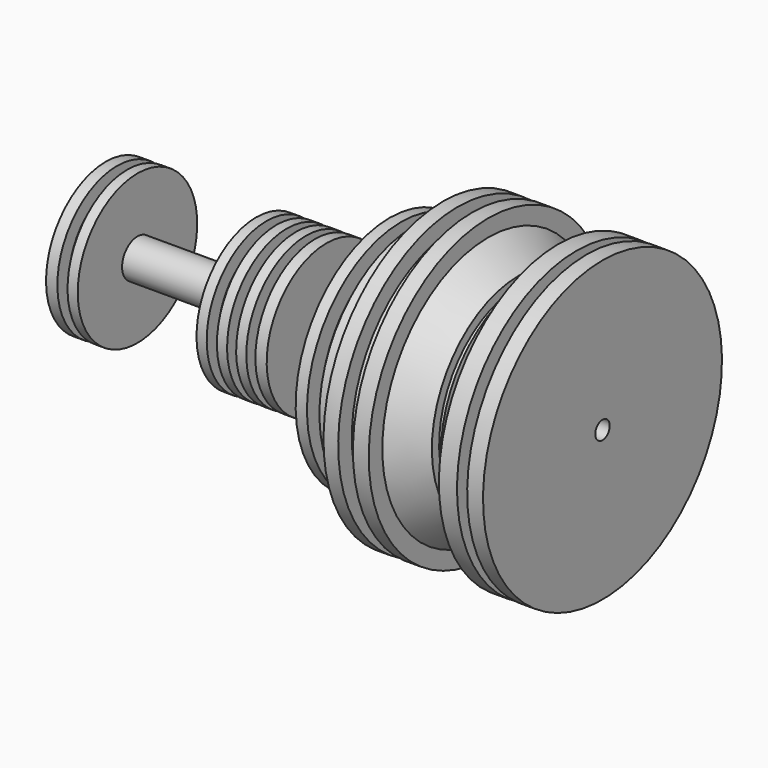
from build123d import *

# Parameters (mm, degrees)
F0_W   = 26.1907838285
F0_H   = 4.2092371732
F0_W_2 = 7.9507762566
F0_W_3 = 3.7415362895
F0_W_4 = 12.6277022064
F0_W_5 = 12.6276984811
F0_W_6 = 49.1077229381
F0_W_7 = 14.0307797119


# Not quite as in the source:
# - ends of sketch curves that miss each other by under 0.0002 mm in the source are joined
# - the program builds the solid bodies; features that only make, move or delete a surface that nothing else refers to are left out


with BuildPart() as f1:
    # F0 (on Front) → F1 (revolve)
    with BuildSketch(Plane.XZ):
        with Locations((-35.0769478828, 2.1046185866)):
            Rectangle(F0_W, F0_H)
        with Locations((-3.9753881283, 2.1046185866)):
            Rectangle(F0_W_2, F0_H)
        with Locations((-62.6708101481, 2.1046185866)):
            Rectangle(F0_W_3, F0_H)
        with Locations((-54.4861909002, 2.1046185866)):
            Rectangle(F0_W_4, F0_H)
        with Locations((-70.8554275334, 2.1046185866)):
            Rectangle(F0_W_5, F0_H)
        with Locations((-101.723138243, 2.1046185866)):
            Rectangle(F0_W_6, F0_H)
        Polygon((-21.9815559685, 44.8984950781), (-21.9815559685, 4.2092371732), (-7.9507762566, 4.2092371732), (-7.9507762566, 44.8984950781), (-12.1600097045, 44.8984950781), (-12.1600097045, 37.4154113233), (-17.3046290874, 37.4154113233), (-17.3046290874, 44.8984950781), align=None)
        with Locations((-14.9661661126, 2.1046185866)):
            Rectangle(F0_W_7, F0_H)
        Polygon((-60.8000420034, 27.1261744201), (-60.8000420034, 4.2092371732), (-48.172339797, 4.2092371732), (-48.172339797, 27.1261744201), (-52.8492666781, 27.1261744201), (-52.8492666781, 21.0461709648), (-56.5908066928, 21.0461709648), (-56.5908066928, 27.1261744201), align=None)
        Polygon((-77.1692767739, 27.1261744201), (-77.1692767739, 4.2092371732), (-64.5415782928, 4.2092371732), (-64.5415782928, 27.1261744201), (-68.7508136034, 27.1261744201), (-68.7508136034, 21.0461709648), (-72.960048914, 21.0461709648), (-72.960048914, 27.1261744201), align=None)
        Polygon((-139.37240839, 27.1261744201), (-139.37240839, 0), (-126.276999712, 0), (-126.276999712, 4.2092371732), (-126.276999712, 27.1261744201), (-130.4862499237, 27.1261744201), (-130.4862499237, 21.0461709648), (-134.6954703331, 21.0461709648), (-134.6954703331, 27.1261744201), align=None)
        Polygon((0, 4.2092371732), (0, 0), (35.0769385695, 0), (35.0769385695, 37.4154113233), (31.3354022801, 37.4154113233), (31.3354022801, 41.1569550633), (18.7077019364, 50.9784966707), (18.7077019364, 57.993888855), (12.1600031853, 57.993888855), (12.1600031853, 50.9784966707), (6.080001127, 50.9784966707), (6.080001127, 57.993888855), (-1.2167e-06, 57.993888855), align=None)
        Polygon((35.0769385695, 37.4154113233), (35.0769385695, 0), (65.9446567297, 0), (65.9446567297, 50.9784966707), (65.9446567297, 57.993888855), (59.396956116, 57.993888855), (59.396956116, 50.9784966707), (55.187728256, 50.9784966707), (55.187728256, 57.993888855), (47.7046445012, 57.993888855), (47.7046445012, 50.9784966707), (35.0769385695, 41.1569550633), align=None)
    revolve(axis=Axis((-53.7846479565, 0, -3.7415372208), (1, 0, 0)))


solid = f1.part
